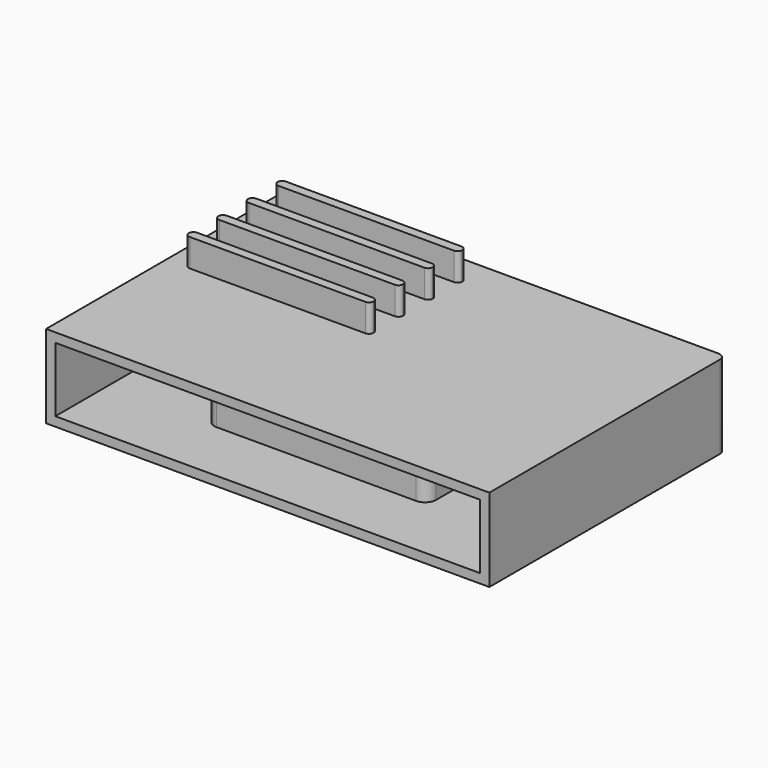
from build123d import *

# Parameters (mm, degrees)
F0_W        = 152.4
F0_H        = 124.46
F1_DEPTH    = 38.1
F2_R        = 7.62
F3_W        = 4.5
F3_H        = 12
F4_DEPTH    = 25.4
F5_W        = 25.4
F5_H        = 9.525
F6_DEPTH    = 38.1
F7_T1_DEPTH = 50.8
F8_W        = 304.8
F8_H        = 57.15
F9_DEPTH    = 101.6
F10_T       = -6.35
F11_R       = 5.08
F12_W       = 127
F12_H       = 6.35
F13_DEPTH   = 19.05
F14_R       = 3.17499


# Not quite as in the source:
# - a fillet or chamfer that OpenCascade refuses, or shapes differently, is made with other operations: its cross-section is extruded or revolved along the edge and cut away or added
# - a fillet or chamfer is up to 0.001 mm smaller than in the source, because OpenCascade refuses the exact size


with BuildPart() as f1:
    # F0 (on Top) → F1 (new body)
    with BuildSketch(Plane.XY):
        Rectangle(F0_W, F0_H)
    extrude(amount=F1_DEPTH)

    # F2
    f2_edges = [f1.edges().sort_by_distance(p)[0] for p in [
        (-76.2, -62.23, 19.05),
        (76.2, -62.23, 19.05),
        (76.2, 62.23, 19.05),
        (-76.2, 62.23, 19.05),
    ]]
    fillet(f2_edges, radius=F2_R)

    # F3 (on face) → F4 (cut)
    with BuildSketch(Plane.YZ.offset(76.2)):
        with Locations((-32.04, 18.7256509207)):
            Rectangle(F3_W, F3_H)
        with Locations((-19.34, 18.7256509207)):
            Rectangle(F3_W, F3_H)
        with Locations((-6.64, 18.7256509207)):
            Rectangle(F3_W, F3_H)
        with Locations((6.06, 18.7256509207)):
            Rectangle(F3_W, F3_H)
        with Locations((18.76, 18.7256509207)):
            Rectangle(F3_W, F3_H)
        with Locations((31.46, 18.7256509207)):
            Rectangle(F3_W, F3_H)
    extrude(amount=-F4_DEPTH, mode=Mode.SUBTRACT)

    # F5 (on face) → F6 (join)
    with BuildSketch(Plane(origin=(-76.2, 0, 0), x_dir=(0, -1, 0), z_dir=(-1, 0, 0))):
        with Locations((1.1544073932, 17.1030452147)):
            Rectangle(F5_W, F5_H)
    extrude(amount=F6_DEPTH)

    # F7: fillet of radius 5.08 on 4 edges, made by hand

    # F7_s2 → F7_t1 (cut)
    with BuildSketch(Plane.YZ.offset(-127)):
        with BuildLine():
            ThreePointArc((-8.7744073932, 21.8655452147), (-12.3665098416, 20.3776476631), (-13.8544073932, 16.7855452147))
            Line((-13.8544073932, 16.7855452147), (-13.8544073932, 21.8655452147))
            Line((-13.8544073932, 21.8655452147), (-8.7744073932, 21.8655452147))
        make_face()
        with BuildLine():
            ThreePointArc((-13.8544073932, 17.4205452147), (-12.3665098416, 13.8284427663), (-8.7744073932, 12.3405452147))
            Line((-8.7744073932, 12.3405452147), (-13.8544073932, 12.3405452147))
            Line((-13.8544073932, 12.3405452147), (-13.8544073932, 17.4205452147))
        make_face()
        with BuildLine():
            ThreePointArc((11.5455926068, 16.7855452147), (10.0576950552, 20.3776476631), (6.4655926068, 21.8655452147))
            Line((6.4655926068, 21.8655452147), (11.5455926068, 21.8655452147))
            Line((11.5455926068, 21.8655452147), (11.5455926068, 16.7855452147))
        make_face()
        with BuildLine():
            ThreePointArc((11.5455926068, 17.4205452147), (10.0576950552, 13.8284427663), (6.4655926068, 12.3405452147))
            Line((6.4655926068, 12.3405452147), (11.5455926068, 12.3405452147))
            Line((11.5455926068, 12.3405452147), (11.5455926068, 17.4205452147))
        make_face()
    extrude(amount=F7_T1_DEPTH, mode=Mode.SUBTRACT)


with BuildPart() as f9:
    # F8 (on Front) → F9 (new body, symmetric)
    with BuildSketch(Plane.XZ):
        with Locations((-2.0108222961, 19.05)):
            Rectangle(F8_W, F8_H)
    extrude(amount=F9_DEPTH, both=True)

    # F10
    f10_openings = [f9.faces().sort_by_distance(p)[0] for p in [
        (-2.010822, -101.6, 19.05),
    ]]
    offset(amount=F10_T, openings=f10_openings)

    # F11
    f11_edges = [f9.edges().sort_by_distance(p)[0] for p in [
        (-154.410822, 101.6, 19.05),
        (150.389178, 101.6, 19.05),
    ]]
    fillet(f11_edges, radius=F11_R)

    # F12 (on face) → F13 (join)
    with BuildSketch(Plane.XY.offset(47.625)):
        with Locations((-77.7289685793, 80.8637710965)):
            Rectangle(F12_W, F12_H)
        with Locations((-77.7289685793, 55.4637710965)):
            Rectangle(F12_W, F12_H)
        with Locations((-77.7289685793, 30.0637710965)):
            Rectangle(F12_W, F12_H)
        with Locations((-77.7289685793, 4.6637710965)):
            Rectangle(F12_W, F12_H)
    extrude(amount=F13_DEPTH)

    # F14 (radius 3.175 in the source; OpenCascade refuses exactly that, so slightly less here)
    f14_edges = [f9.edges().sort_by_distance(p)[0] for p in [
        (-141.228969, 84.038771, 57.15),
        (-141.228969, 77.688771, 57.15),
        (-141.228969, 58.638771, 57.15),
        (-141.228969, 33.238771, 57.15),
        (-141.228969, 7.838771, 57.15),
        (-141.228969, 1.488771, 57.15),
        (-14.228969, 77.688771, 57.15),
        (-14.228969, 84.038771, 57.15),
        (-14.228969, 58.638771, 57.15),
        (-14.228969, 52.288771, 57.15),
        (-14.228969, 33.238771, 57.15),
        (-14.228969, 26.888771, 57.15),
        (-14.228969, 7.838771, 57.15),
        (-14.228969, 1.488771, 57.15),
        (-141.228969, 52.288771, 57.15),
        (-141.228969, 26.888771, 57.15),
    ]]
    fillet(f14_edges, radius=F14_R)


solid = Compound([f1.part, f9.part])
